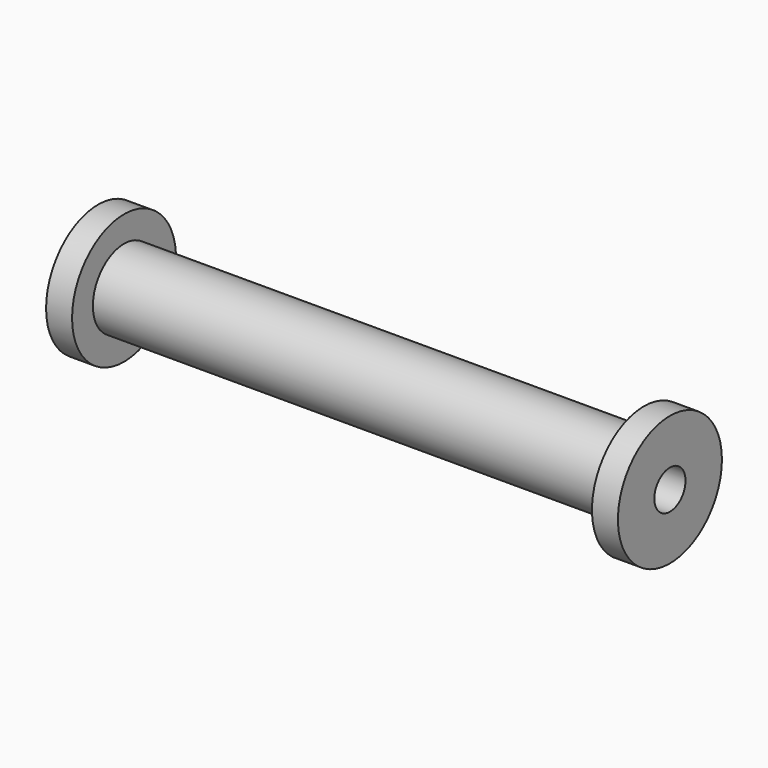
from build123d import *

# Parameters (mm, degrees)
F0_R     = 3
F1_DEPTH = 40
F2_R     = 5
F2_R_2   = 3
F3_DEPTH = 2
F4_R     = 5
F4_R_2   = 3
F5_DEPTH = 2
F6_R     = 1.5
F7_DEPTH = 44


with BuildPart() as f1:
    # F0 (on Right) → F1 (new body)
    with BuildSketch(Plane.YZ):
        with Locations((-6.2035736628, 2.2626414429)):
            Circle(F0_R)
    extrude(amount=F1_DEPTH)

    # F2 (on face) → F3 (join)
    with BuildSketch(Plane.YZ.offset(40)):
        with Locations((-6.2035736628, 2.2626414429)):
            Circle(F2_R)
        with Locations((-6.2035736628, 2.2626414429)):
            Circle(F2_R_2, mode=Mode.SUBTRACT)
        with Locations((-6.2035736628, 2.2626414429)):
            Circle(F2_R_2)
    extrude(amount=F3_DEPTH)

    # F4 (on face) → F5 (join)
    with BuildSketch(Plane(origin=(0, 0, 0), x_dir=(0, -1, 0), z_dir=(-1, 0, 0))):
        with Locations((6.2035736628, 2.2626414429)):
            Circle(F4_R)
        with Locations((6.2035736628, 2.2626414429)):
            Circle(F4_R_2, mode=Mode.SUBTRACT)
        with Locations((6.2035736628, 2.2626414429)):
            Circle(F4_R_2)
    extrude(amount=F5_DEPTH)

    # F6 (on face) → F7 (cut)
    with BuildSketch(Plane.YZ.offset(42)):
        with Locations((-6.2035736628, 2.2626414429)):
            Circle(F6_R)
    extrude(amount=-F7_DEPTH, mode=Mode.SUBTRACT)


solid = f1.part
